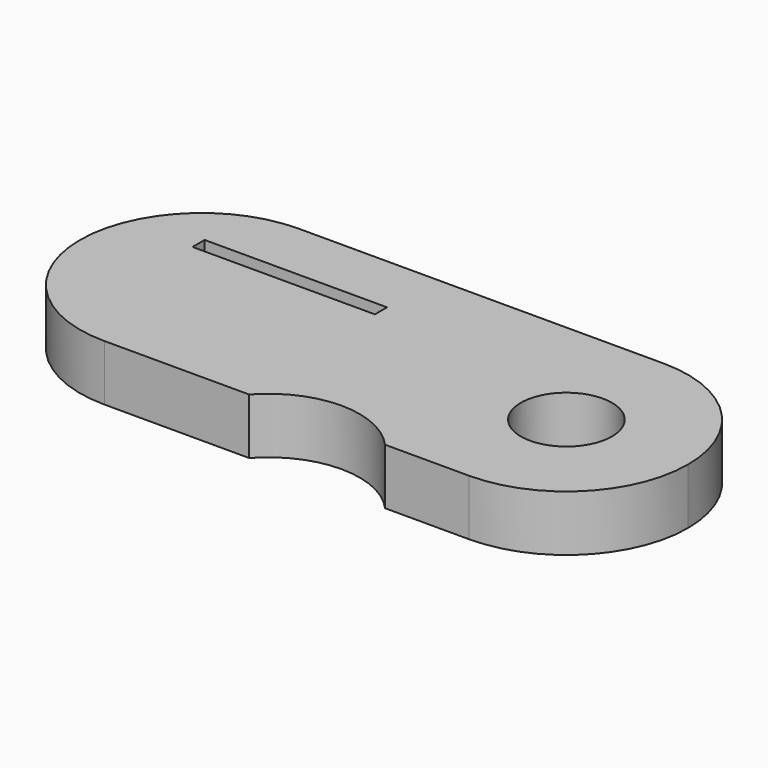
from build123d import *

# Parameters (mm, degrees)
F1_DEPTH = 5.842
F2_R     = 4.7625
F3_DEPTH = 25.4
F4_W     = 19.05
F4_H     = 1.5875
F5_DEPTH = 25.4
F7_DEPTH = 25.4


# Not quite as in the source:
# - a feature names something its author has since deleted; it is built from what else it names


with BuildPart() as f1:
    # F0 (on Top) → F1 (new body)
    with BuildSketch(Plane.XY):
        with BuildLine():
            Line((-38.1, 25.4), (-38.1, 0))
            ThreePointArc((-38.1, 0), (-29.1197438789, 3.7197438789), (-25.4, 12.7))
            ThreePointArc((-25.4, 12.7), (-29.1197438789, 21.6802561211), (-38.1, 25.4))
        make_face()
        with BuildLine():
            ThreePointArc((0, 25.4), (-12.7, 12.7), (0, 0))
            Line((0, 0), (0, 25.4))
        make_face()
        with BuildLine():
            Line((-38.1, 0), (0, 0))
            ThreePointArc((0, 0), (-12.7, 12.7), (0, 25.4))
            Line((0, 25.4), (-38.1, 25.4))
            ThreePointArc((-38.1, 25.4), (-29.1197438789, 21.6802561211), (-25.4, 12.7))
            ThreePointArc((-25.4, 12.7), (-29.1197438789, 3.7197438789), (-38.1, 0))
        make_face()
        with BuildLine():
            Line((0, 25.4), (0, 0))
            ThreePointArc((0, 0), (8.9802561211, 3.7197438789), (12.7, 12.7))
            ThreePointArc((12.7, 12.7), (8.9802561211, 21.6802561211), (0, 25.4))
        make_face()
        with BuildLine():
            ThreePointArc((-38.1, 25.4), (-50.8, 12.7), (-38.1, 0))
            Line((-38.1, 0), (-38.1, 25.4))
        make_face()
    extrude(amount=F1_DEPTH)

    # F2 (on face) → F3 (cut)
    with BuildSketch(Plane.XY.offset(5.842)):
        with Locations((0, 12.7)):
            Circle(F2_R)
    extrude(amount=-F3_DEPTH, mode=Mode.SUBTRACT)

    # F4 (on face) → F5 (cut)
    with BuildSketch(Plane.XY.offset(5.842)):
        with Locations((-33.3375, 18.25625)):
            Rectangle(F4_W, F4_H)
    extrude(amount=-F5_DEPTH, mode=Mode.SUBTRACT)

    # F6 (on face) → F7 (cut)
    with BuildSketch(Plane(origin=(0, 0, 0), x_dir=(1, 0, 0), z_dir=(0, 0, -1))):
        with BuildLine():
            Line((-8.7754841714, 0), (-22.9745158286, 0))
            ThreePointArc((-22.9745158286, 0), (-15.875, -3.175), (-8.7754841714, 0))
        make_face()
    extrude(amount=-F7_DEPTH, mode=Mode.SUBTRACT)


solid = f1.part
